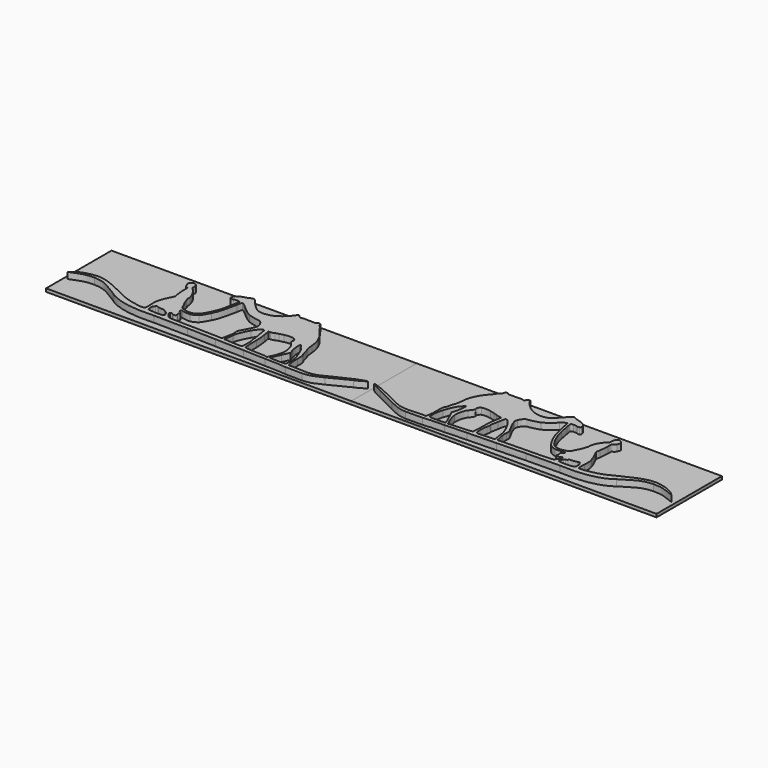
from build123d import *

# Parameters (mm, degrees)
F1_DEPTH = 2
F2_W     = 96.982617
F2_H     = 25.9708038449
F3_DEPTH = 1


# Not quite as in the source:
# - ends of sketch curves that miss each other by under 0.0002 mm in the source are joined


with BuildPart() as f1:
    # F0 (on Top) → F1 (new body)
    with BuildSketch(Plane.XY):
        with BuildLine():
            add(Edge.make_bspline(
                [(26.691874, -11.927583), (25.657716, -11.753169), (23.579804, -11.652992), (20.017703, -11.605818)],
                knots=[0, 0, 0, 0, 1, 1, 1, 1], degree=3))
            add(Edge.make_bspline(
                [(32.047701, -11.997616), (30.612274, -12.006111), (27.693789, -11.992423), (26.691874, -11.927583)],
                knots=[0, 0, 0, 0, 1, 1, 1, 1], degree=3))
            add(Edge.make_bspline(
                [(37.871114, -10.161981), (33.930318, -12.127275), (33.41182, -11.769755), (32.047701, -11.997616)],
                knots=[0, 0, 0, 0, 1, 1, 1, 1], degree=3))
            add(Edge.make_bspline(
                [(44.295003, -6.903307), (42.859271, -7.568347), (41.245168, -8.479321), (37.871114, -10.161981)],
                knots=[0, 0, 0, 0, 1, 1, 1, 1], degree=3))
            add(Edge.make_bspline(
                [(47.491308, -5.210222), (45.586999, -6.316471), (44.862402, -6.734321), (44.295003, -6.903307)],
                knots=[0, 0, 0, 0, 1, 1, 1, 1], degree=3))
            add(Edge.make_bspline(
                [(39.722405, -8.326128), (43.61465, -6.350352), (46.92664, -5.022), (47.491308, -5.210222)],
                knots=[0, 0, 0, 0, 1, 1, 1, 1], degree=3))
            add(Edge.make_bspline(
                [(34.083413, -10.674818), (35.419472, -10.469436), (35.868807, -10.282283), (39.722405, -8.326128)],
                knots=[0, 0, 0, 0, 1, 1, 1, 1], degree=3))
            add(Edge.make_bspline(
                [(30.829752, -10.767511), (32.09838, -10.859366), (33.061325, -10.831931), (34.083413, -10.674818)],
                knots=[0, 0, 0, 0, 1, 1, 1, 1], degree=3))
            add(Edge.make_bspline(
                [(27.835475, -10.636241), (28.491272, -10.636805), (29.838697, -10.695759), (30.829752, -10.767511)],
                knots=[0, 0, 0, 0, 1, 1, 1, 1], degree=3))
            Line((27.835475, -10.636241), (26.643115, -10.635394))
            Line((26.643115, -10.635394), (26.432574, -9.614794))
            add(Edge.make_bspline(
                [(26.243736, -6.546612), (26.231798, -7.672783), (26.316778, -9.053462), (26.432574, -9.614794)],
                knots=[0, 0, 0, 0, 1, 1, 1, 1], degree=3))
            add(Edge.make_bspline(
                [(25.941163, -3.965806), (26.21957, -4.42361), (26.262366, -4.788653), (26.243736, -6.546612)],
                knots=[0, 0, 0, 0, 1, 1, 1, 1], degree=3))
            add(Edge.make_bspline(
                [(25.506753, -2.676301), (25.567326, -3.092255), (25.762813, -3.672532), (25.941163, -3.965806)],
                knots=[0, 0, 0, 0, 1, 1, 1, 1], degree=3))
            add(Edge.make_bspline(
                [(25.086357, -1.303954), (25.257, -1.64279), (25.446176, -2.260348), (25.506753, -2.676301)],
                knots=[0, 0, 0, 0, 1, 1, 1, 1], degree=3))
            add(Edge.make_bspline(
                [(24.605044, 1.263363), (24.717103, -0.014918), (24.883104, -0.900359), (25.086357, -1.303954)],
                knots=[0, 0, 0, 0, 1, 1, 1, 1], degree=3))
            add(Edge.make_bspline(
                [(23.863274, 4.531575), (24.337653, 3.436908), (24.462861, 2.885252), (24.605044, 1.263363)],
                knots=[0, 0, 0, 0, 1, 1, 1, 1], degree=3))
            add(Edge.make_bspline(
                [(21.322066, 8.374536), (22.477729, 7.111947), (23.253369, 5.938978), (23.863274, 4.531575)],
                knots=[0, 0, 0, 0, 1, 1, 1, 1], degree=3))
            add(Edge.make_bspline(
                [(20.329696, 9.734855), (20.480886, 9.417804), (20.927454, 8.805659), (21.322066, 8.374536)],
                knots=[0, 0, 0, 0, 1, 1, 1, 1], degree=3))
            add(Edge.make_bspline(
                [(19.66083, 10.490819), (19.877514, 10.392089), (20.178502, 10.051907), (20.329696, 9.734855)],
                knots=[0, 0, 0, 0, 1, 1, 1, 1], degree=3))
            add(Edge.make_bspline(
                [(19.266859, 10.974237), (19.266859, 10.807083), (19.444145, 10.589546), (19.66083, 10.490819)],
                knots=[0, 0, 0, 0, 1, 1, 1, 1], degree=3))
            add(Edge.make_bspline(
                [(18.079443, 11.4049), (18.499601, 11.911161), (19.266859, 11.632887), (19.266859, 10.974237)],
                knots=[0, 0, 0, 0, 1, 1, 1, 1], degree=3))
            add(Edge.make_bspline(
                [(15.702776, 11.226798), (17.567461, 11.143867), (17.882389, 11.167466), (18.079443, 11.4049)],
                knots=[0, 0, 0, 0, 1, 1, 1, 1], degree=3))
            add(Edge.make_bspline(
                [(13.254905, 11.136069), (13.456338, 11.261867), (14.251544, 11.291339), (15.702776, 11.226798)],
                knots=[0, 0, 0, 0, 1, 1, 1, 1], degree=3))
            add(Edge.make_bspline(
                [(12.509505, 11.481029), (12.881336, 11.039134), (13.006749, 10.981095), (13.254905, 11.136069)],
                knots=[0, 0, 0, 0, 1, 1, 1, 1], degree=3))
            add(Edge.make_bspline(
                [(11.373995, 11.553462), (11.499087, 12.174475), (11.950222, 12.145696), (12.509505, 11.481029)],
                knots=[0, 0, 0, 0, 1, 1, 1, 1], degree=3))
            add(Edge.make_bspline(
                [(8.232086, 8.272724), (9.444577, 9.072652), (11.255092, 10.963166), (11.373995, 11.553462)],
                knots=[0, 0, 0, 0, 1, 1, 1, 1], degree=3))
            add(Edge.make_bspline(
                [(2.555208, 7.396924), (3.935566, 6.789079), (6.60823, 7.201406), (8.232086, 8.272724)],
                knots=[0, 0, 0, 0, 1, 1, 1, 1], degree=3))
            add(Edge.make_bspline(
                [(-1.028548, 10.636705), (0.141613, 9.188961), (1.714307, 7.767219), (2.555208, 7.396924)],
                knots=[0, 0, 0, 0, 1, 1, 1, 1], degree=3))
            add(Edge.make_bspline(
                [(-3.636776, 11.341174), (-2.305118, 12.035271), (-2.118141, 11.98477), (-1.028548, 10.636705)],
                knots=[0, 0, 0, 0, 1, 1, 1, 1], degree=3))
            add(Edge.make_bspline(
                [(-4.608944, 11.011186), (-4.422454, 11.011186), (-3.984979, 11.15968), (-3.636776, 11.341174)],
                knots=[0, 0, 0, 0, 1, 1, 1, 1], degree=3))
            add(Edge.make_bspline(
                [(-6.921202, 9.852124), (-6.75539, 10.169466), (-5.076213, 11.011186), (-4.608944, 11.011186)],
                knots=[0, 0, 0, 0, 1, 1, 1, 1], degree=3))
            add(Edge.make_bspline(
                [(-7.166509, 9.080484), (-7.10608, 9.362325), (-6.995691, 9.709565), (-6.921202, 9.852124)],
                knots=[0, 0, 0, 0, 1, 1, 1, 1], degree=3))
            add(Edge.make_bspline(
                [(-6.886714, 8.390501), (-7.214493, 8.539848), (-7.258931, 8.649432), (-7.166509, 9.080484)],
                knots=[0, 0, 0, 0, 1, 1, 1, 1], degree=3))
            add(Edge.make_bspline(
                [(-6.087449, 8.416014), (-6.386103, 8.267955), (-6.60259, 8.261043), (-6.886714, 8.390501)],
                knots=[0, 0, 0, 0, 1, 1, 1, 1], degree=3))
            add(Edge.make_bspline(
                [(-4.885298, 8.546917), (-5.325088, 8.586956), (-5.860167, 8.528686), (-6.087449, 8.416014)],
                knots=[0, 0, 0, 0, 1, 1, 1, 1], degree=3))
            add(Edge.make_bspline(
                [(-4.327069, 6.705908), (-3.962556, 8.444245), (-3.968378, 8.463444), (-4.885298, 8.546917)],
                knots=[0, 0, 0, 0, 1, 1, 1, 1], degree=3))
            add(Edge.make_bspline(
                [(-4.912555, 3.651953), (-4.690339, 4.7034), (-4.455945, 6.091288), (-4.327069, 6.705908)],
                knots=[0, 0, 0, 0, 1, 1, 1, 1], degree=3))
            add(Edge.make_bspline(
                [(-6.268639, -0.251482), (-5.481324, 1.374279), (-5.21201, 2.235045), (-4.912555, 3.651953)],
                knots=[0, 0, 0, 0, 1, 1, 1, 1], degree=3))
            add(Edge.make_bspline(
                [(-10.499816, -3.83024), (-8.533613, -3.850137), (-7.649067, -3.101972), (-6.268639, -0.251482)],
                knots=[0, 0, 0, 0, 1, 1, 1, 1], degree=3))
            add(Edge.make_bspline(
                [(-12.34829, -3.439656), (-11.799726, -3.649742), (-10.967913, -3.825505), (-10.499816, -3.83024)],
                knots=[0, 0, 0, 0, 1, 1, 1, 1], degree=3))
            add(Edge.make_bspline(
                [(-13.451093, -2.542252), (-13.360039, -2.987451), (-13.209782, -3.109721), (-12.34829, -3.439656)],
                knots=[0, 0, 0, 0, 1, 1, 1, 1], degree=3))
            add(Edge.make_bspline(
                [(-14.050104, -1.28163), (-13.778626, -1.691484), (-13.509073, -2.258765), (-13.451093, -2.542252)],
                knots=[0, 0, 0, 0, 1, 1, 1, 1], degree=3))
            add(Edge.make_bspline(
                [(-14.75295, 0.3986), (-14.637863, -0.115671), (-14.321582, -0.871773), (-14.050104, -1.28163)],
                knots=[0, 0, 0, 0, 1, 1, 1, 1], degree=3))
            add(Edge.make_bspline(
                [(-15.128334, 1.333633), (-15.036962, 1.333633), (-14.86804, 0.912868), (-14.75295, 0.3986)],
                knots=[0, 0, 0, 0, 1, 1, 1, 1], degree=3))
            add(Edge.make_bspline(
                [(-15.193482, 1.651808), (-15.249021, 1.476813), (-15.2197, 1.333633), (-15.128334, 1.333633)],
                knots=[0, 0, 0, 0, 1, 1, 1, 1], degree=3))
            add(Edge.make_bspline(
                [(-17.152237, 6.09825), (-15.989244, 5.026951), (-14.904089, 2.563609), (-15.193482, 1.651808)],
                knots=[0, 0, 0, 0, 1, 1, 1, 1], degree=3))
            add(Edge.make_bspline(
                [(-17.8911, 7.307744), (-17.963013, 6.931562), (-17.842225, 6.733837), (-17.152237, 6.09825)],
                knots=[0, 0, 0, 0, 1, 1, 1, 1], degree=3))
            add(Edge.make_bspline(
                [(-19.222681, 9.066898), (-18.522251, 9.314957), (-17.712019, 8.244556), (-17.8911, 7.307744)],
                knots=[0, 0, 0, 0, 1, 1, 1, 1], degree=3))
            add(Edge.make_bspline(
                [(-20.277608, 8.060329), (-20.277608, 8.321992), (-19.658782, 8.912449), (-19.222681, 9.066898)],
                knots=[0, 0, 0, 0, 1, 1, 1, 1], degree=3))
            add(Edge.make_bspline(
                [(-19.925522, 7.088288), (-20.119169, 7.500254), (-20.277608, 7.93767), (-20.277608, 8.060329)],
                knots=[0, 0, 0, 0, 1, 1, 1, 1], degree=3))
            add(Edge.make_bspline(
                [(-19.200448, 6.339262), (-19.478854, 6.339262), (-19.662722, 6.529203), (-19.925522, 7.088288)],
                knots=[0, 0, 0, 0, 1, 1, 1, 1], degree=3))
            add(Edge.make_bspline(
                [(-18.840967, 4.795859), (-18.827929, 6.286238), (-18.840403, 6.339262), (-19.200448, 6.339262)],
                knots=[0, 0, 0, 0, 1, 1, 1, 1], degree=3))
            add(Edge.make_bspline(
                [(-18.619956, 1.914238), (-18.748943, 2.650259), (-18.848395, 3.946988), (-18.840967, 4.795859)],
                knots=[0, 0, 0, 0, 1, 1, 1, 1], degree=3))
            Line((-18.619956, 1.914238), (-18.385435, 0.576019))
            Line((-18.385435, 0.576019), (-19.052072, -0.755429))
            add(Edge.make_bspline(
                [(-20.10558, -3.290454), (-19.892804, -2.628487), (-19.418724, -1.487728), (-19.052072, -0.755429)],
                knots=[0, 0, 0, 0, 1, 1, 1, 1], degree=3))
            add(Edge.make_bspline(
                [(-20.374295, -6.514081), (-20.482146, -4.67023), (-20.458704, -4.389043), (-20.10558, -3.290454)],
                knots=[0, 0, 0, 0, 1, 1, 1, 1], degree=3))
            add(Edge.make_bspline(
                [(-20.454158, -8.772733), (-20.310425, -8.599548), (-20.28853, -7.980327), (-20.374295, -6.514081)],
                knots=[0, 0, 0, 0, 1, 1, 1, 1], degree=3))
            add(Edge.make_bspline(
                [(-22.551261, -8.840043), (-22.189734, -8.932138), (-20.686305, -9.052455), (-20.454158, -8.772733)],
                knots=[0, 0, 0, 0, 1, 1, 1, 1], degree=3))
            add(Edge.make_bspline(
                [(-27.851372, -7.454809), (-25.010235, -8.592865), (-24.285655, -8.433511), (-22.551261, -8.840043)],
                knots=[0, 0, 0, 0, 1, 1, 1, 1], degree=3))
            add(Edge.make_bspline(
                [(-40.243704, -2.862128), (-35.903304, -2.819157), (-30.692511, -6.316754), (-27.851372, -7.454809)],
                knots=[0, 0, 0, 0, 1, 1, 1, 1], degree=3))
            add(Edge.make_bspline(
                [(-47.491309, -5.80712), (-45.485531, -3.773141), (-43.09291, -3.184699), (-40.243704, -2.862128)],
                knots=[0, 0, 0, 0, 1, 1, 1, 1], degree=3))
            add(Edge.make_bspline(
                [(-40.288849, -3.99858), (-43.5054, -4.014046), (-44.016327, -4.459926), (-47.491309, -5.80712)],
                knots=[0, 0, 0, 0, 1, 1, 1, 1], degree=3))
            add(Edge.make_bspline(
                [(-31.477007, -7.686528), (-35.436133, -5.43208), (-36.292785, -4.216749), (-40.288849, -3.99858)],
                knots=[0, 0, 0, 0, 1, 1, 1, 1], degree=3))
            add(Edge.make_bspline(
                [(-15.973183, -10.693086), (-24.157862, -11.196565), (-28.989867, -9.618706), (-31.477007, -7.686528)],
                knots=[0, 0, 0, 0, 1, 1, 1, 1], degree=3))
            add(Edge.make_bspline(
                [(-5.294509, -10.84232), (-6.276677, -10.750372), (-11.082388, -10.748692), (-15.973183, -10.693086)],
                knots=[0, 0, 0, 0, 1, 1, 1, 1], degree=3))
            add(Edge.make_bspline(
                [(3.832837, -11.100928), (-0.205035, -11.050642), (-4.312342, -10.934268), (-5.294509, -10.84232)],
                knots=[0, 0, 0, 0, 1, 1, 1, 1], degree=3))
            add(Edge.make_bspline(
                [(13.009823, -11.364837), (12.000356, -11.269974), (7.870711, -11.151215), (3.832837, -11.100928)],
                knots=[0, 0, 0, 0, 1, 1, 1, 1], degree=3))
            add(Edge.make_bspline(
                [(20.017703, -11.605818), (17.172838, -11.568142), (14.019292, -11.4597), (13.009823, -11.364837)],
                knots=[0, 0, 0, 0, 1, 1, 1, 1], degree=3))
        make_face()
        with BuildLine():
            add(Edge.make_bspline(
                [(-15.470111, -9.21405), (-14.129716, -9.144886), (-13.955574, -8.971759), (-14.29439, -8.342658)],
                knots=[0, 0, 0, 0, 1, 1, 1, 1], degree=3))
            add(Edge.make_bspline(
                [(-16.506109, -9.238135), (-16.315324, -9.221625), (-16.141181, -9.248661), (-15.470111, -9.21405)],
                knots=[0, 0, 0, 0, 1, 1, 1, 1], degree=3))
            add(Edge.make_bspline(
                [(-16.936207, -9.25535), (-16.760078, -9.263055), (-16.67816, -9.242932), (-16.506109, -9.238135)],
                knots=[0, 0, 0, 0, 1, 1, 1, 1], degree=3))
            add(Edge.make_bspline(
                [(-18.115007, -9.124591), (-17.668774, -9.162448), (-17.26376, -9.241025), (-16.936207, -9.25535)],
                knots=[0, 0, 0, 0, 1, 1, 1, 1], degree=3))
            add(Edge.make_bspline(
                [(-18.885155, -9.031692), (-18.62404, -9.101071), (-18.323882, -9.106867), (-18.115007, -9.124591)],
                knots=[0, 0, 0, 0, 1, 1, 1, 1], degree=3))
            add(Edge.make_bspline(
                [(-19.411485, -8.106494), (-19.365051, -8.825873), (-19.312566, -8.918128), (-18.885155, -9.031692)],
                knots=[0, 0, 0, 0, 1, 1, 1, 1], degree=3))
            add(Edge.make_bspline(
                [(-19.228281, -7.033118), (-19.378665, -7.208827), (-19.444522, -7.594681), (-19.411485, -8.106494)],
                knots=[0, 0, 0, 0, 1, 1, 1, 1], degree=3))
            add(Edge.make_bspline(
                [(-18.891821, -6.471696), (-18.94774, -6.629603), (-19.099147, -6.882242), (-19.228281, -7.033118)],
                knots=[0, 0, 0, 0, 1, 1, 1, 1], degree=3))
            add(Edge.make_bspline(
                [(-18.094636, -6.429984), (-18.73306, -6.204734), (-18.798493, -6.20816), (-18.891821, -6.471696)],
                knots=[0, 0, 0, 0, 1, 1, 1, 1], degree=3))
            add(Edge.make_bspline(
                [(-16.591704, -6.675371), (-17.035789, -6.675371), (-17.712107, -6.564945), (-18.094636, -6.429984)],
                knots=[0, 0, 0, 0, 1, 1, 1, 1], degree=3))
            add(Edge.make_bspline(
                [(-15.605687, -7.009081), (-15.746511, -6.745952), (-15.95505, -6.675371), (-16.591704, -6.675371)],
                knots=[0, 0, 0, 0, 1, 1, 1, 1], degree=3))
            add(Edge.make_bspline(
                [(-15.015829, -7.342789), (-15.246433, -7.274523), (-15.501251, -7.204224), (-15.605687, -7.009081)],
                knots=[0, 0, 0, 0, 1, 1, 1, 1], degree=3))
            add(Edge.make_bspline(
                [(-14.610188, -7.639371), (-14.750833, -7.46351), (-14.825786, -7.399048), (-15.015829, -7.342789)],
                knots=[0, 0, 0, 0, 1, 1, 1, 1], degree=3))
            add(Edge.make_bspline(
                [(-14.29439, -8.342658), (-14.347402, -8.213205), (-14.427347, -7.985333), (-14.610188, -7.639371)],
                knots=[0, 0, 0, 0, 1, 1, 1, 1], degree=3))
        make_face(mode=Mode.SUBTRACT)
        with BuildLine():
            add(Edge.make_bspline(
                [(0.742975, -9.573361), (1.147831, -9.604699), (1.578172, -9.579683), (2.697197, -9.621694)],
                knots=[0, 0, 0, 0, 1, 1, 1, 1], degree=3))
            add(Edge.make_bspline(
                [(-0.46479, -9.550958), (-0.084444, -9.579787), (0.250598, -9.553216), (0.742975, -9.573361)],
                knots=[0, 0, 0, 0, 1, 1, 1, 1], degree=3))
            add(Edge.make_bspline(
                [(-6.053492, -9.439582), (-3.015895, -9.480741), (-0.691538, -9.520616), (-0.46479, -9.550958)],
                knots=[0, 0, 0, 0, 1, 1, 1, 1], degree=3))
            add(Edge.make_bspline(
                [(-12.161484, -9.254983), (-11.839686, -9.315353), (-9.09109, -9.39842), (-6.053492, -9.439582)],
                knots=[0, 0, 0, 0, 1, 1, 1, 1], degree=3))
            add(Edge.make_bspline(
                [(-13.207995, -8.452541), (-12.860368, -8.974384), (-12.602267, -9.172292), (-12.161484, -9.254983)],
                knots=[0, 0, 0, 0, 1, 1, 1, 1], degree=3))
            add(Edge.make_bspline(
                [(-13.903949, -7.532784), (-13.754273, -7.860176), (-13.473033, -8.102509), (-13.207995, -8.452541)],
                knots=[0, 0, 0, 0, 1, 1, 1, 1], degree=3))
            add(Edge.make_bspline(
                [(-13.887693, -7.05492), (-13.971099, -7.236778), (-13.952365, -7.394312), (-13.903949, -7.532784)],
                knots=[0, 0, 0, 0, 1, 1, 1, 1], degree=3))
            add(Edge.make_bspline(
                [(-13.118697, -7.056613), (-13.575251, -6.786922), (-13.619543, -6.786829), (-13.887693, -7.05492)],
                knots=[0, 0, 0, 0, 1, 1, 1, 1], degree=3))
            add(Edge.make_bspline(
                [(-11.933618, -6.510889), (-11.515531, -7.292094), (-12.192404, -7.603789), (-13.118697, -7.056613)],
                knots=[0, 0, 0, 0, 1, 1, 1, 1], degree=3))
            add(Edge.make_bspline(
                [(-11.936892, -5.926937), (-12.076465, -6.095113), (-12.075624, -6.24556), (-11.933618, -6.510889)],
                knots=[0, 0, 0, 0, 1, 1, 1, 1], degree=3))
            add(Edge.make_bspline(
                [(-12.467907, -4.949997), (-12.018445, -5.067534), (-11.703909, -5.646211), (-11.936892, -5.926937)],
                knots=[0, 0, 0, 0, 1, 1, 1, 1], degree=3))
            add(Edge.make_bspline(
                [(-12.087739, -4.31301), (-12.848404, -4.141148), (-12.682599, -4.70336), (-12.467907, -4.949997)],
                knots=[0, 0, 0, 0, 1, 1, 1, 1], degree=3))
            add(Edge.make_bspline(
                [(-9.484417, -4.538787), (-10.050733, -4.713415), (-11.796418, -4.359777), (-12.087739, -4.31301)],
                knots=[0, 0, 0, 0, 1, 1, 1, 1], degree=3))
            add(Edge.make_bspline(
                [(-7.506711, -3.570232), (-8.012919, -4.028056), (-8.867575, -4.458879), (-9.484417, -4.538787)],
                knots=[0, 0, 0, 0, 1, 1, 1, 1], degree=3))
            add(Edge.make_bspline(
                [(-5.693724, -0.728807), (-6.253808, -1.872106), (-7.061026, -3.254101), (-7.506711, -3.570232)],
                knots=[0, 0, 0, 0, 1, 1, 1, 1], degree=3))
            add(Edge.make_bspline(
                [(-3.571029, 6.60905), (-4.309653, 2.691746), (-4.809062, 1.077042), (-5.693724, -0.728807)],
                knots=[0, 0, 0, 0, 1, 1, 1, 1], degree=3))
            add(Edge.make_bspline(
                [(-3.054306, 8.226539), (-3.312776, 8.266933), (-3.27108, 8.19984), (-3.571029, 6.60905)],
                knots=[0, 0, 0, 0, 1, 1, 1, 1], degree=3))
            add(Edge.make_bspline(
                [(-1.499622, 7.20267), (-1.96536, 7.631659), (-2.647446, 8.162954), (-3.054306, 8.226539)],
                knots=[0, 0, 0, 0, 1, 1, 1, 1], degree=3))
            add(Edge.make_bspline(
                [(2.181261, 4.420303), (1.333084, 4.795698), (0.108982, 5.720992), (-1.499622, 7.20267)],
                knots=[0, 0, 0, 0, 1, 1, 1, 1], degree=3))
            add(Edge.make_bspline(
                [(6.000529, 3.50274), (5.330147, 3.50274), (2.977218, 4.068022), (2.181261, 4.420303)],
                knots=[0, 0, 0, 0, 1, 1, 1, 1], degree=3))
            add(Edge.make_bspline(
                [(7.491247, 1.806423), (7.159822, 2.674245), (6.431745, 3.50274), (6.000529, 3.50274)],
                knots=[0, 0, 0, 0, 1, 1, 1, 1], degree=3))
            add(Edge.make_bspline(
                [(7.443102, 0.069583), (7.763823, 1.018924), (7.765728, 1.087699), (7.491247, 1.806423)],
                knots=[0, 0, 0, 0, 1, 1, 1, 1], degree=3))
            add(Edge.make_bspline(
                [(6.408256, -2.170308), (6.793757, -1.482033), (7.259438, -0.474082), (7.443102, 0.069583)],
                knots=[0, 0, 0, 0, 1, 1, 1, 1], degree=3))
            add(Edge.make_bspline(
                [(5.32516, -5.239935), (5.206658, -4.291462), (5.183589, -4.356839), (6.408256, -2.170308)],
                knots=[0, 0, 0, 0, 1, 1, 1, 1], degree=3))
            add(Edge.make_bspline(
                [(5.187503, -7.272668), (5.343654, -6.54377), (5.394415, -5.794219), (5.32516, -5.239935)],
                knots=[0, 0, 0, 0, 1, 1, 1, 1], degree=3))
            add(Edge.make_bspline(
                [(4.835965, -9.062711), (4.893261, -8.713258), (5.051452, -7.907739), (5.187503, -7.272668)],
                knots=[0, 0, 0, 0, 1, 1, 1, 1], degree=3))
            Line((4.835965, -9.062711), (4.731788, -9.698078))
            Line((4.731788, -9.698078), (2.697197, -9.621694))
        make_face(mode=Mode.SUBTRACT)
        with BuildLine():
            add(Edge.make_bspline(
                [(11.251985, -9.689718), (11.507162, -9.212912), (11.466575, -6.48471), (11.194414, -5.819763)],
                knots=[0, 0, 0, 0, 1, 1, 1, 1], degree=3))
            add(Edge.make_bspline(
                [(10.04229, -9.986294), (10.912677, -10.008251), (11.107004, -9.960612), (11.251985, -9.689718)],
                knots=[0, 0, 0, 0, 1, 1, 1, 1], degree=3))
            add(Edge.make_bspline(
                [(5.522168, -9.668823), (5.599108, -9.748926), (8.38238, -9.94441), (10.04229, -9.986294)],
                knots=[0, 0, 0, 0, 1, 1, 1, 1], degree=3))
            add(Edge.make_bspline(
                [(5.678912, -8.427344), (5.553873, -9.06973), (5.483337, -9.628397), (5.522168, -9.668823)],
                knots=[0, 0, 0, 0, 1, 1, 1, 1], degree=3))
            add(Edge.make_bspline(
                [(5.912383, -6.703398), (5.909024, -7.00918), (5.803947, -7.784953), (5.678912, -8.427344)],
                knots=[0, 0, 0, 0, 1, 1, 1, 1], degree=3))
            add(Edge.make_bspline(
                [(7.807104, -1.945682), (6.754988, -3.641041), (5.923121, -5.729889), (5.912383, -6.703398)],
                knots=[0, 0, 0, 0, 1, 1, 1, 1], degree=3))
            add(Edge.make_bspline(
                [(9.934278, 0.332509), (9.406943, 0.332509), (8.852232, -0.261583), (7.807104, -1.945682)],
                knots=[0, 0, 0, 0, 1, 1, 1, 1], degree=3))
            add(Edge.make_bspline(
                [(10.678927, -2.086877), (10.337441, 0.21344), (10.300791, 0.332509), (9.934278, 0.332509)],
                knots=[0, 0, 0, 0, 1, 1, 1, 1], degree=3))
            add(Edge.make_bspline(
                [(11.081308, -4.229494), (11.049883, -4.064516), (10.828784, -3.096347), (10.678927, -2.086877)],
                knots=[0, 0, 0, 0, 1, 1, 1, 1], degree=3))
            add(Edge.make_bspline(
                [(11.040781, -4.675806), (11.123037, -4.402093), (11.112731, -4.394476), (11.081308, -4.229494)],
                knots=[0, 0, 0, 0, 1, 1, 1, 1], degree=3))
            add(Edge.make_bspline(
                [(11.194414, -5.819763), (10.976485, -4.838417), (11.019295, -4.747302), (11.040781, -4.675806)],
                knots=[0, 0, 0, 0, 1, 1, 1, 1], degree=3))
        make_face(mode=Mode.SUBTRACT)
        with BuildLine():
            add(Edge.make_bspline(
                [(25.679591, -10.26274), (25.941237, -9.292897), (25.76152, -7.175866), (25.286566, -5.632892)],
                knots=[0, 0, 0, 0, 1, 1, 1, 1], degree=3))
            add(Edge.make_bspline(
                [(24.221894, -10.598409), (25.447432, -10.596716), (25.598921, -10.561768), (25.679591, -10.26274)],
                knots=[0, 0, 0, 0, 1, 1, 1, 1], degree=3))
            add(Edge.make_bspline(
                [(21.711877, -10.548704), (22.340169, -10.577118), (23.469675, -10.599487), (24.221894, -10.598409)],
                knots=[0, 0, 0, 0, 1, 1, 1, 1], degree=3))
            Line((21.711877, -10.548704), (20.569526, -10.49704))
            Line((20.569526, -10.49704), (20.681086, -10.046182))
            add(Edge.make_bspline(
                [(21.850011, -7.392633), (21.268458, -8.604114), (20.742444, -9.798207), (20.681086, -10.046182)],
                knots=[0, 0, 0, 0, 1, 1, 1, 1], degree=3))
            Line((21.850011, -7.392633), (22.907376, -5.189948))
            Line((22.907376, -5.189948), (22.505379, -3.924051))
            add(Edge.make_bspline(
                [(22.262408, -0.168054), (21.933571, -0.168054), (22.092417, -2.623627), (22.505379, -3.924051)],
                knots=[0, 0, 0, 0, 1, 1, 1, 1], degree=3))
            add(Edge.make_bspline(
                [(22.701292, -0.757814), (22.54737, -0.433448), (22.349871, -0.168054), (22.262408, -0.168054)],
                knots=[0, 0, 0, 0, 1, 1, 1, 1], degree=3))
            add(Edge.make_bspline(
                [(23.294286, -1.515157), (23.122062, -1.422986), (22.855216, -1.082183), (22.701292, -0.757814)],
                knots=[0, 0, 0, 0, 1, 1, 1, 1], degree=3))
            add(Edge.make_bspline(
                [(25.286566, -5.632892), (24.712627, -3.768372), (23.737126, -1.752159), (23.294286, -1.515157)],
                knots=[0, 0, 0, 0, 1, 1, 1, 1], degree=3))
        make_face(mode=Mode.SUBTRACT)
        with BuildLine():
            add(Edge.make_bspline(
                [(19.905, -10.304452), (19.880842, -10.18974), (19.996451, -9.893017), (20.161893, -9.645068)],
                knots=[0, 0, 0, 0, 1, 1, 1, 1], degree=3))
            add(Edge.make_bspline(
                [(19.239802, -10.430343), (19.413549, -10.604093), (19.946831, -10.503165), (19.905, -10.304452)],
                knots=[0, 0, 0, 0, 1, 1, 1, 1], degree=3))
            add(Edge.make_bspline(
                [(14.624938, -10.190403), (16.289115, -10.180808), (19.138391, -10.328935), (19.239802, -10.430343)],
                knots=[0, 0, 0, 0, 1, 1, 1, 1], degree=3))
            add(Edge.make_bspline(
                [(12.845547, -10.013309), (13.152435, -10.114593), (13.953162, -10.194284), (14.624938, -10.190403)],
                knots=[0, 0, 0, 0, 1, 1, 1, 1], degree=3))
            Line((12.845547, -10.013309), (12.287565, -9.829159))
            Line((12.287565, -9.829159), (12.186496, -8.460833))
            add(Edge.make_bspline(
                [(12.108292, -5.257111), (12.095705, -6.26658), (12.130898, -7.708253), (12.186496, -8.460833)],
                knots=[0, 0, 0, 0, 1, 1, 1, 1], degree=3))
            add(Edge.make_bspline(
                [(11.804607, -1.586317), (12.014902, -2.768275), (12.123021, -4.075153), (12.108292, -5.257111)],
                knots=[0, 0, 0, 0, 1, 1, 1, 1], degree=3))
            add(Edge.make_bspline(
                [(11.493093, 0.272596), (11.484824, 0.25967), (11.625001, -0.576847), (11.804607, -1.586317)],
                knots=[0, 0, 0, 0, 1, 1, 1, 1], degree=3))
            add(Edge.make_bspline(
                [(12.179096, 0.371439), (11.810068, 0.330009), (11.501365, 0.285528), (11.493093, 0.272596)],
                knots=[0, 0, 0, 0, 1, 1, 1, 1], degree=3))
            add(Edge.make_bspline(
                [(13.263648, 0.669133), (13.036174, 0.546832), (12.548124, 0.412866), (12.179096, 0.371439)],
                knots=[0, 0, 0, 0, 1, 1, 1, 1], degree=3))
            add(Edge.make_bspline(
                [(14.344658, 1.036767), (13.977577, 0.956869), (13.491125, 0.791434), (13.263648, 0.669133)],
                knots=[0, 0, 0, 0, 1, 1, 1, 1], degree=3))
            add(Edge.make_bspline(
                [(15.679493, 1.35443), (15.312412, 1.259612), (14.711736, 1.116664), (14.344658, 1.036767)],
                knots=[0, 0, 0, 0, 1, 1, 1, 1], degree=3))
            add(Edge.make_bspline(
                [(18.699968, 1.410725), (18.119933, 1.641936), (16.689315, 1.615271), (15.679493, 1.35443)],
                knots=[0, 0, 0, 0, 1, 1, 1, 1], degree=3))
            add(Edge.make_bspline(
                [(19.33017, -0.07688), (19.539452, 0.468498), (19.229755, 1.199544), (18.699968, 1.410725)],
                knots=[0, 0, 0, 0, 1, 1, 1, 1], degree=3))
            add(Edge.make_bspline(
                [(20.390129, -1.858119), (19.683111, -1.086944), (19.232899, -0.330369), (19.33017, -0.07688)],
                knots=[0, 0, 0, 0, 1, 1, 1, 1], degree=3))
            add(Edge.make_bspline(
                [(21.370786, -5.896008), (21.497574, -4.654394), (20.972813, -2.493678), (20.390129, -1.858119)],
                knots=[0, 0, 0, 0, 1, 1, 1, 1], degree=3))
            add(Edge.make_bspline(
                [(20.161893, -9.645068), (20.623741, -8.952884), (21.260183, -6.979132), (21.370786, -5.896008)],
                knots=[0, 0, 0, 0, 1, 1, 1, 1], degree=3))
        make_face(mode=Mode.SUBTRACT)
    extrude(amount=F1_DEPTH)

    # F2 (on face) → F3 (join)
    with BuildSketch(Plane(origin=(0, 0, 0), x_dir=(1, 0, 0), z_dir=(0, 0, -1))):
        with Locations((-5e-07, 0.0122140776)):
            Rectangle(F2_W, F2_H)
    extrude(amount=F3_DEPTH)


with BuildPart() as f4_1:
    # F4: instance of F1
    add(f1.part.mirror(Plane(origin=(48.491308, -0.0122140776, -0.5), x_dir=(0, 1, 0), z_dir=(1, 0, 0))))


solid = Compound([f1.part, f4_1.part])
